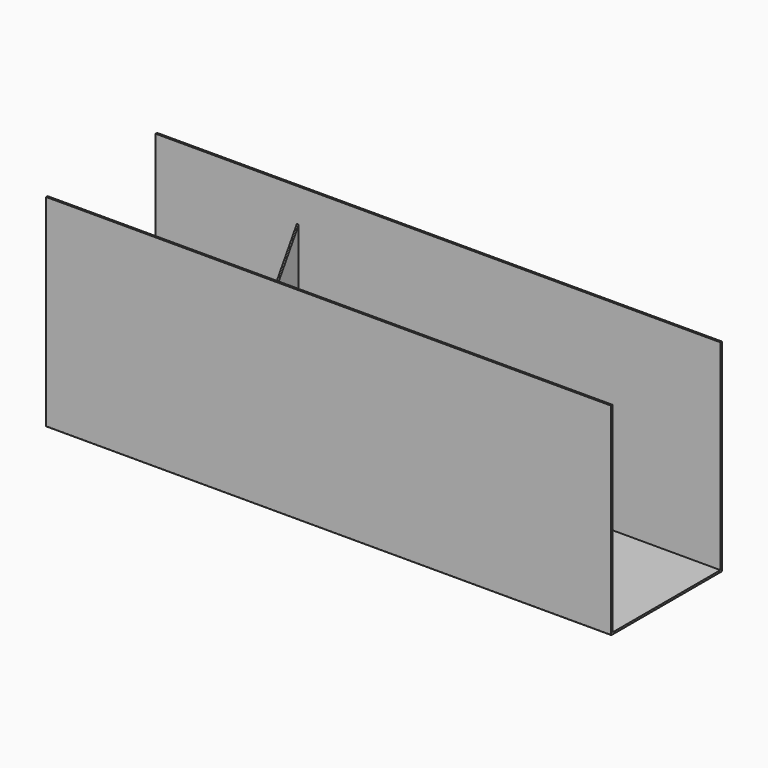
from build123d import *

# Parameters (mm, degrees)
F1_DEPTH = 1200
F4_DEPTH = 4
F7_DEPTH = 4
F8_W     = 1200
F8_H     = 230
F9_DEPTH = 4
F10_R    = 2


# Not quite as in the source:
# - a feature names something its author has since deleted; it is built from what else it names


with BuildPart() as f1:
    # F0 (on Right) → F1 (new body)
    with BuildSketch(Plane.YZ):
        Polygon((-295, 0), (0, 0), (0, 430), (-4, 430), (-4, 4), (-291, 4), (-291, 430), (-295, 430), align=None)
    extrude(amount=F1_DEPTH)

    # F6 (on offset) → F7 (join)
    with BuildSketch(Plane.YZ.offset(894)):
        Polygon((-291, 359), (-291, 4), (-69, 4), align=None)
    extrude(amount=F7_DEPTH)



with BuildPart() as f4:
    # F3 (on offset) → F4 (new body)
    with BuildSketch(Plane.YZ.offset(300)):
        Polygon((-226, 4), (-4, 4), (-4, 359), align=None)
    extrude(amount=F4_DEPTH)


with BuildPart() as f1_1:
    add(f1.part)

    add(f4.part)  # F9 merges F4
    # F8 (on Top) → F9 (join)
    with BuildSketch(Plane.XY):
        with Locations((600, -115)):
            Rectangle(F8_W, F8_H)
    extrude(amount=F9_DEPTH)

    # F10
    f10_edges = [f1_1.edges().sort_by_distance(p)[0] for p in [
        (600, 0, 0),
        (600, -295, 0),
    ]]
    fillet(f10_edges, radius=F10_R)


solid = f1_1.part
